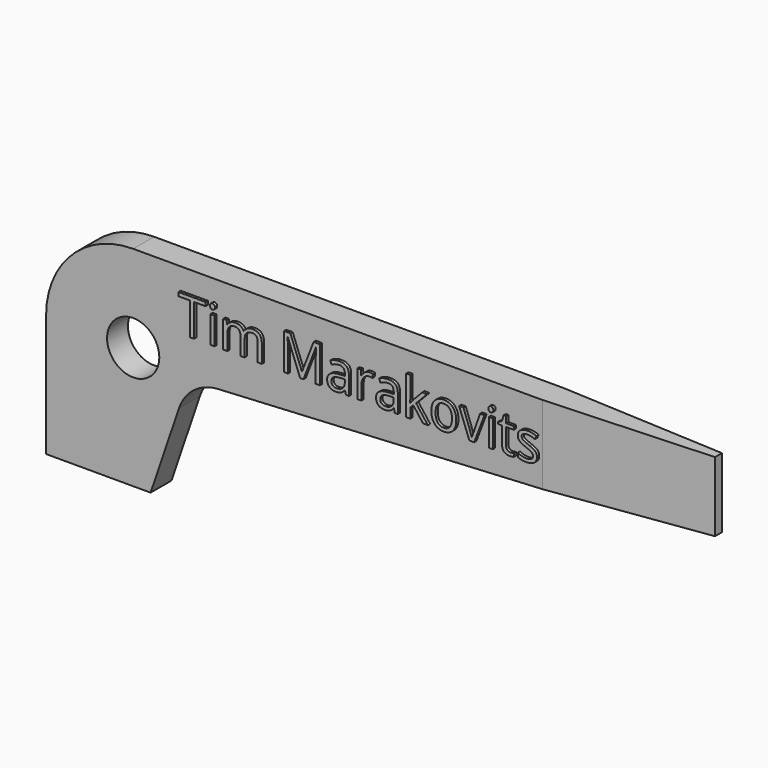
from build123d import *

# Parameters (mm, degrees)
F1_DEPTH     = 2.38125
F2_R         = 2.38125
F3_DEPTH     = 2.38225
F5_DEPTH     = 19.051
F6_TEXT_SIZE = 4.6173745849
F7_DEPTH     = 0.254


# Not quite as in the source:
# - Text() gives the source's letters only with a copy of the font that has no kerning and outlines rounded to 1/6400 em; it was checked with that copy


with BuildPart() as f1:
    # F0 (on Front) → F1 (new body)
    with BuildSketch(Plane.XZ):
        with BuildLine():
            Line((60.325, 19.05), (7.9375, 19.05))
            ThreePointArc((7.9375, 19.05), (2.3248399243, 16.7251600757), (0, 11.1125))
            Line((0, 11.1125), (0, 0))
            Line((0, 0), (9.525, 0))
            Line((9.525, 0), (12.1173647876, 7.6271664624))
            ThreePointArc((12.1173647876, 7.6271664624), (13.4786145605, 9.5135918491), (15.6631963617, 10.3130942181))
            Line((15.6631963617, 10.3130942181), (60.325, 12.7))
            Line((60.325, 12.7), (60.325, 19.05))
        make_face()
    extrude(amount=F1_DEPTH)

    # F2 (on face) → F3 (cut, through all)
    with BuildSketch(Plane.XZ.offset(2.38125)):
        with Locations((7.9375, 11.1125)):
            Circle(F2_R)
    extrude(amount=-F3_DEPTH, mode=Mode.SUBTRACT)

    # F4 (on face) → F5 (cut, through all)
    with BuildSketch(Plane.XY.offset(19.05)):
        Polygon((60.325, -2.38125), (60.325, -1.5875), (45.24375, -2.38125), align=None)
        Polygon((60.325, 0), (45.24375, 0), (60.325, -0.79375), align=None)
    extrude(amount=-F5_DEPTH, mode=Mode.SUBTRACT)

    # F6 (on face) → F7 (join)
    with BuildSketch(Plane.XZ.offset(2.38125)):
        with Locations((12.22375, 13.7989975574)):
            Text('Tim Marakovits', F6_TEXT_SIZE, font='Open Sans', text_align=(TextAlign.LEFT, TextAlign.BOTTOM))
    extrude(amount=F7_DEPTH)


solid = f1.part
